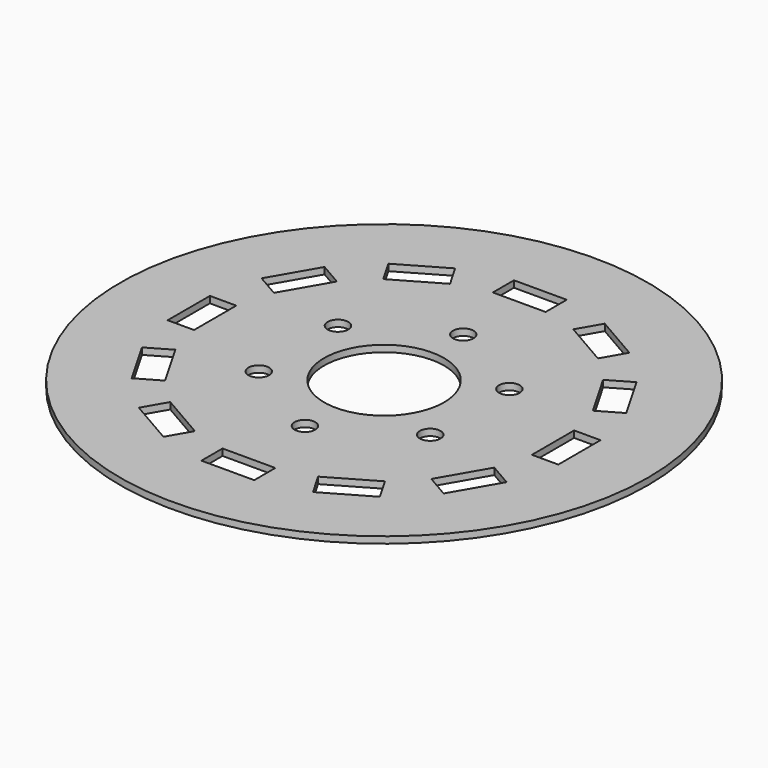
from build123d import *

# Parameters (mm, degrees)
F0_R            = 63.5
F0_R_2          = 14.4272
F1_DEPTH        = 1.5875
F2_W            = 12.7
F2_H            = 6.35
F3_DEPTH        = 1.5885
F3_COPIES_COUNT = 12
F4_R            = 2.4892
F5_DEPTH        = 1.5885
F5_COPIES_COUNT = 6


# Not quite as in the source:
# - a pattern or mirror of a feature is missing from the dataset's text; its kind, count and spacing are read off the source's solid


with BuildPart() as f1:
    # F0 (on Top) → F1 (new body)
    with BuildSketch(Plane.XY):
        Circle(F0_R)
        Circle(F0_R_2, mode=Mode.SUBTRACT)
    extrude(amount=F1_DEPTH)

    # F2 (on face) → F3 (cut, through all)
    with BuildSketch(Plane.XY.offset(1.5875)):
        with Locations((0, 43.815)):
            Rectangle(F2_W, F2_H)
    f3 = extrude(amount=-F3_DEPTH, mode=Mode.SUBTRACT)

    # F3_copies: F3 ×12 about axis
    f3_copies_axis = Axis((0, 0, 0), (0, 0, 1))
    for i in range(1, F3_COPIES_COUNT):
        add(f3.rotate(f3_copies_axis, i * 360 / F3_COPIES_COUNT), mode=Mode.SUBTRACT)

    # F4 (on face) → F5 (cut, through all)
    with BuildSketch(Plane.XY.offset(1.5875)):
        with Locations((0, 23.8125)):
            Circle(F4_R)
    f5 = extrude(amount=-F5_DEPTH, mode=Mode.SUBTRACT)

    # F5_copies: F5 ×6 about axis
    f5_copies_axis = Axis((0, 0, 0), (0, 0, 1))
    for i in range(1, F5_COPIES_COUNT):
        add(f5.rotate(f5_copies_axis, i * 360 / F5_COPIES_COUNT), mode=Mode.SUBTRACT)


solid = f1.part
